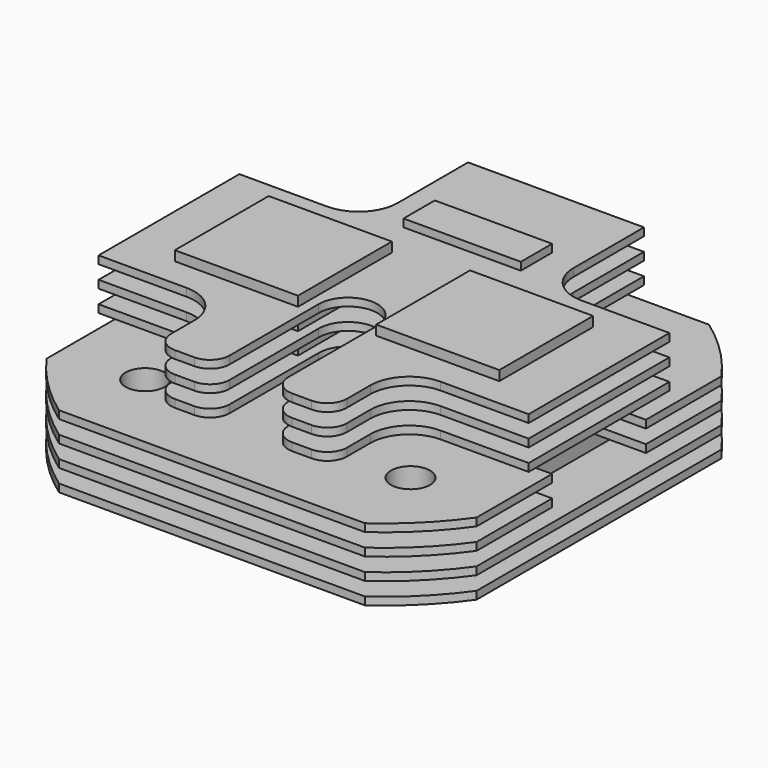
from build123d import *

# Parameters (mm, degrees)
F0_W        = 220
F0_H        = 220
F1_DEPTH    = 4
F2_W        = 166
F2_H        = 166
F3_DEPTH    = 7
F5_DEPTH    = 2
F6_W        = 220
F6_H        = 220
F6_W_2      = 166
F6_H_2      = 166
F7_DEPTH    = 4
F8_W        = 166
F8_H        = 166
F9_DEPTH    = 7
F10_W       = 220
F10_H       = 220
F10_W_2     = 166
F10_H_2     = 166
F11_DEPTH   = 4
F12_W       = 166
F12_H       = 60
F13_DEPTH   = 49
F14_W       = 60
F14_H       = 49
F14_H_2     = 11
F15_DEPTH   = 30
F16_W       = 166
F16_H       = 53
F17_DEPTH   = 7
F18_W       = 60
F18_H       = 60
F19_DEPTH   = 30
F20_W       = 166
F20_H       = 53
F17_FACE1_W = 166
F17_FACE1_H = 53
F21_DEPTH   = 4
F22_W       = 40
F22_H       = 38
F23_DEPTH   = 60
F24_W       = 60
F24_H       = 20
F25_DEPTH   = 7
F26_W       = 220
F26_H       = 220
F26_W_2     = 60
F26_H_2     = 20
F27_DEPTH   = 4
F28_W       = 60
F28_H       = 20
F29_DEPTH   = 7
F30_W       = 220
F30_H       = 220
F30_W_2     = 60
F30_H_2     = 20
F31_DEPTH   = 4
F32_W       = 60
F32_H       = 20
F33_DEPTH   = 7
F34_W       = 220
F34_H       = 220
F34_W_2     = 60
F34_H_2     = 20
F35_DEPTH   = 4
F36_W       = 60
F36_H       = 20
F37_DEPTH   = 4
F38_R       = 185
F39_DEPTH   = 70
F4_R        = 10
F40_DEPTH   = 100
F43_DEPTH   = 135
F45_DEPTH   = 135


with BuildPart() as f1:
    # F0 (on Top) → F1 (new body)
    with BuildSketch(Plane.XY):
        Rectangle(F0_W, F0_H)
    extrude(amount=F1_DEPTH)

    # F2 (on face) → F3 (join)
    with BuildSketch(Plane.XY.offset(4)):
        Rectangle(F2_W, F2_H)
    extrude(amount=F3_DEPTH)

    # F4 (on face) → F5 (join)
    with BuildSketch(Plane(origin=(0, 0, 0), x_dir=(1, 0, 0), z_dir=(0, 0, -1))):
        with BuildLine():
            ThreePointArc((-56.5685424949, 56.5685424949), (-30.6146745892, -73.9103626009), (80, 0))
            ThreePointArc((80, 0), (30.6146745892, 73.9103626009), (-56.5685424949, 56.5685424949))
        make_face()
    extrude(amount=F5_DEPTH)

    # F6 (on face) → F7 (join)
    with BuildSketch(Plane.XY.offset(11)):
        Rectangle(F6_W, F6_H)
        Rectangle(F6_W_2, F6_H_2, mode=Mode.SUBTRACT)
        Rectangle(F6_W_2, F6_H_2)
    extrude(amount=F7_DEPTH)

    # F8 (on face) → F9 (join)
    with BuildSketch(Plane.XY.offset(15)):
        Rectangle(F8_W, F8_H)
    extrude(amount=F9_DEPTH)

    # F10 (on face) → F11 (join)
    with BuildSketch(Plane.XY.offset(22)):
        Rectangle(F10_W, F10_H)
        Rectangle(F10_W_2, F10_H_2, mode=Mode.SUBTRACT)
        Rectangle(F10_W_2, F10_H_2)
    extrude(amount=F11_DEPTH)

    # F12 (on face) → F13 (join)
    with BuildSketch(Plane.XY.offset(26)):
        Rectangle(F12_W, F12_H)
    extrude(amount=F13_DEPTH)

    # F14 (on face) → F15 (cut)
    with BuildSketch(Plane.YZ.offset(83)):
        with Locations((0, 50.5)):
            Rectangle(F14_W, F14_H)
        with Locations((0, 20.5)):
            Rectangle(F14_W, F14_H_2)
    extrude(amount=F15_DEPTH, mode=Mode.SUBTRACT)

    # F16 (on face) → F17 (join)
    with BuildSketch(Plane.XY.offset(26)):
        with Locations((0, -56.5)):
            Rectangle(F16_W, F16_H)
        with Locations((0, 56.5)):
            Rectangle(F16_W, F16_H)
    extrude(amount=F17_DEPTH)

    # F18 (on face) → F19 (cut)
    with BuildSketch(Plane(origin=(-83, 0, 0), x_dir=(0, -1, 0), z_dir=(-1, 0, 0))):
        with Locations((0, 45)):
            Rectangle(F18_W, F18_H)
    extrude(amount=F19_DEPTH, mode=Mode.SUBTRACT)

    # F20 (on face) + F17_face1 (on face) → F21 (join)
    with BuildSketch(Plane.XY.offset(33)):
        Polygon((-110, 110), (-110, 30), (-83, 30), (-83, 83), (83, 83), (83, 30), (110, 30), (110, 110), align=None)
        with Locations((0, 56.5)):
            Rectangle(F20_W, F20_H)
        Polygon((-83, -83), (-83, -30), (-110, -30), (-110, -110), (110, -110), (110, -30), (83, -30), (83, -83), align=None)
    with BuildSketch(Plane(origin=(0, 56.5, 33), x_dir=(1, 0, 0), z_dir=(0, 0, 1))):
        with Locations((0, -113)):
            Rectangle(F17_FACE1_W, F17_FACE1_H)
    extrude(amount=F21_DEPTH)

    # F22 (on face) → F23 (cut)
    with BuildSketch(Plane.XZ.offset(30)):
        with Locations((0, 56)):
            Rectangle(F22_W, F22_H)
    extrude(amount=-F23_DEPTH, mode=Mode.SUBTRACT)

    # F24 (on face) → F25 (join)
    with BuildSketch(Plane.XY.offset(37)):
        with Locations((0, 60)):
            Rectangle(F24_W, F24_H)
    extrude(amount=F25_DEPTH)

    # F26 (on face) → F27 (join)
    with BuildSketch(Plane.XY.offset(44)):
        Rectangle(F26_W, F26_H)
        with Locations((0, 60)):
            Rectangle(F26_W_2, F26_H_2, mode=Mode.SUBTRACT)
        with Locations((0, 60)):
            Rectangle(F26_W_2, F26_H_2)
    extrude(amount=F27_DEPTH)

    # F28 (on face) → F29 (join)
    with BuildSketch(Plane.XY.offset(48)):
        with Locations((0, 60)):
            Rectangle(F28_W, F28_H)
    extrude(amount=F29_DEPTH)

    # F30 (on face) → F31 (join)
    with BuildSketch(Plane.XY.offset(55)):
        Rectangle(F30_W, F30_H)
        with Locations((0, 60)):
            Rectangle(F30_W_2, F30_H_2, mode=Mode.SUBTRACT)
        with Locations((0, 60)):
            Rectangle(F30_W_2, F30_H_2)
    extrude(amount=F31_DEPTH)

    # F32 (on face) → F33 (join)
    with BuildSketch(Plane.XY.offset(59)):
        with Locations((0, 60)):
            Rectangle(F32_W, F32_H)
    extrude(amount=F33_DEPTH)

    # F34 (on face) → F35 (join)
    with BuildSketch(Plane.XY.offset(66)):
        Rectangle(F34_W, F34_H)
        with Locations((0, 60)):
            Rectangle(F34_W_2, F34_H_2, mode=Mode.SUBTRACT)
        with Locations((0, 60)):
            Rectangle(F34_W_2, F34_H_2)
    extrude(amount=F35_DEPTH)

    # F36 (on face) → F37 (join)
    with BuildSketch(Plane.XY.offset(70)):
        with Locations((0, 60)):
            Rectangle(F36_W, F36_H)
    extrude(amount=F37_DEPTH)

    # F38 (on face) → F39 (cut)
    with BuildSketch(Plane(origin=(0, 0, 0), x_dir=(1, 0, 0), z_dir=(0, 0, -1))):
        Circle(F38_R)
        with BuildLine():
            ThreePointArc((110, 78.2623792125), (128.5982114961, 41.0791918129), (135, 0))
            ThreePointArc((135, 0), (128.5982114961, -41.0791918129), (110, -78.2623792125))
            Line((110, -78.2623792125), (110, -110))
            Line((110, -110), (78.2623792125, -110))
            ThreePointArc((78.2623792125, -110), (0, -135), (-78.2623792125, -110))
            Line((-78.2623792125, -110), (-110, -110))
            Line((-110, -110), (-110, -78.2623792125))
            ThreePointArc((-110, -78.2623792125), (-135, 0), (-110, 78.2623792125))
            Line((-110, 78.2623792125), (-110, 110))
            Line((-110, 110), (-78.2623792125, 110))
            ThreePointArc((-78.2623792125, 110), (0, 135), (78.2623792125, 110))
            Line((78.2623792125, 110), (110, 110))
            Line((110, 110), (110, 78.2623792125))
        make_face(mode=Mode.SUBTRACT)
        with BuildLine():
            ThreePointArc((78.2623792125, 110), (95.4594154602, 95.4594154602), (110, 78.2623792125))
            Line((110, 78.2623792125), (110, 110))
            Line((110, 110), (78.2623792125, 110))
        make_face()
        with BuildLine():
            Line((110, -110), (110, -78.2623792125))
            ThreePointArc((110, -78.2623792125), (95.4594154602, -95.4594154602), (78.2623792125, -110))
            Line((78.2623792125, -110), (110, -110))
        make_face()
        with BuildLine():
            ThreePointArc((-110, 78.2623792125), (-95.4594154602, 95.4594154602), (-78.2623792125, 110))
            Line((-78.2623792125, 110), (-110, 110))
            Line((-110, 110), (-110, 78.2623792125))
        make_face()
        with BuildLine():
            Line((-110, -110), (-78.2623792125, -110))
            ThreePointArc((-78.2623792125, -110), (-95.4594154602, -95.4594154602), (-110, -78.2623792125))
            Line((-110, -78.2623792125), (-110, -110))
        make_face()
    extrude(amount=-F39_DEPTH, mode=Mode.SUBTRACT)

    # F4 (on face) → F40 (cut)
    with BuildSketch(Plane(origin=(0, 0, 0), x_dir=(1, 0, 0), z_dir=(0, 0, -1))):
        with BuildLine():
            ThreePointArc((-74.9533188058, 74.9533188058), (-74.9533188058, 60.811183182), (-60.811183182, 60.811183182))
            Line((-60.811183182, 60.811183182), (-74.9533188058, 74.9533188058))
        make_face()
        with BuildLine():
            Line((-74.9533188058, 74.9533188058), (-60.811183182, 60.811183182))
            ThreePointArc((-60.811183182, 60.811183182), (-58.6434556688, 64.0554166703), (-57.8822509939, 67.8822509939))
            ThreePointArc((-57.8822509939, 67.8822509939), (-64.0554166703, 77.121046319), (-74.9533188058, 74.9533188058))
        make_face()
        with Locations((-67.8822509939, -67.8822509939)):
            Circle(F4_R)
        with Locations((67.8822509939, 67.8822509939)):
            Circle(F4_R)
        with Locations((67.8822509939, -67.8822509939)):
            Circle(F4_R)
    extrude(amount=-F40_DEPTH, mode=Mode.SUBTRACT)

    # F42 (on offset) → F43 (cut)
    with BuildSketch(Plane.XY.offset(175)):
        with BuildLine():
            Line((145, -145), (145, -45))
            Line((145, -45), (65, -45))
            ThreePointArc((65, -45), (50.8578643763, -50.8578643763), (45, -65))
            Line((45, -65), (45, -80))
            ThreePointArc((45, -80), (42.0710678119, -87.0710678119), (35, -90))
            Line((35, -90), (25, -90))
            ThreePointArc((25, -90), (17.9289321881, -87.0710678119), (15, -80))
            Line((15, -80), (15, -23))
            ThreePointArc((15, -23), (0, -8), (-15, -23))
            Line((-15, -23), (-15, -80))
            ThreePointArc((-15, -80), (-17.9289321881, -87.0710678119), (-25, -90))
            Line((-25, -90), (-35, -90))
            ThreePointArc((-35, -90), (-42.0710678119, -87.0710678119), (-45, -80))
            Line((-45, -80), (-45, -65))
            ThreePointArc((-45, -65), (-50.8578643763, -50.8578643763), (-65, -45))
            Line((-65, -45), (-145, -45))
            Line((-145, -45), (-145, -145))
            Line((-145, -145), (45, -145))
            Line((45, -145), (145, -145))
        make_face()
    extrude(amount=-F43_DEPTH, mode=Mode.SUBTRACT)

    # F44 (on offset) → F45 (cut)
    with BuildSketch(Plane.XY.offset(175)):
        with BuildLine():
            Line((132.7324633664, 45), (132.7324633664, 137.0121001288))
            Line((132.7324633664, 137.0121001288), (45, 137.0121001288))
            Line((45, 137.0121001288), (45, 65))
            ThreePointArc((45, 65), (50.8578643763, 50.8578643763), (65, 45))
            Line((65, 45), (132.7324633664, 45))
        make_face()
        with BuildLine():
            Line((-45, 65), (-45, 137.0121001288))
            Line((-45, 137.0121001288), (-153.8187099461, 137.0121001288))
            Line((-153.8187099461, 137.0121001288), (-153.8187099461, 45))
            Line((-153.8187099461, 45), (-65, 45))
            ThreePointArc((-65, 45), (-50.8578643763, 50.8578643763), (-45, 65))
        make_face()
    extrude(amount=-F45_DEPTH, mode=Mode.SUBTRACT)


solid = f1.part
